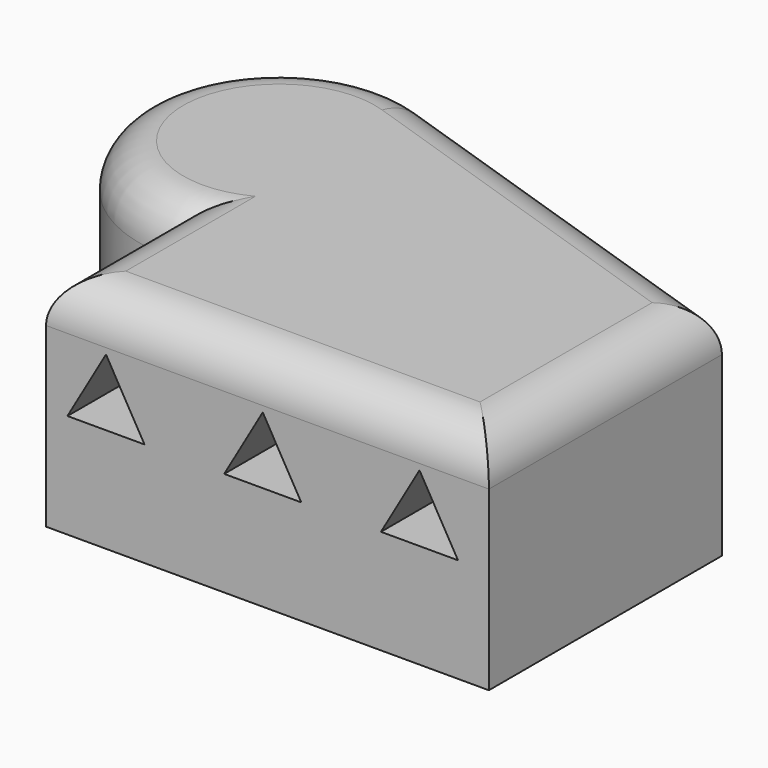
from build123d import *

# Parameters (mm, degrees)
F1_DEPTH = 25
F4_DEPTH = 25
F5_DEPTH = 23.7095438224
F6_R     = 5


# Not quite as in the source:
# - the program builds the solid bodies; features that only make, move or delete a surface that nothing else refers to are left out


with BuildPart() as f1:
    # F0 (on Top) → F1 (new body)
    with BuildSketch(Plane.XY):
        with BuildLine():
            ThreePointArc((-24.4463197887, 8.4633977604), (-29.1204506303, 19.7477478306), (-17.8361005601, 15.073616989))
            Line((-17.8361005601, 15.073616989), (-8.6304908186, 15.073616989))
            ThreePointArc((-8.6304908186, 15.073616989), (-11.6154192696, 24.3206942504), (-19.4435108685, 30.0773614855))
            ThreePointArc((-19.4435108685, 30.0773614855), (-40.0578075922, 17.607762717), (-24.4463197887, -0.7422119811))
            Line((-24.4463197887, -0.7422119811), (-24.4463197887, 8.4633977604))
        make_face()
        with BuildLine():
            Line((-17.8361005601, 15.073616989), (-24.4463197887, 15.073616989))
            Line((-24.4463197887, 15.073616989), (-24.4463197887, 8.4633977604))
            ThreePointArc((-24.4463197887, 8.4633977604), (-19.772188947, 10.3994861473), (-17.8361005601, 15.073616989))
        make_face()
        with BuildLine():
            Line((-24.4463197887, 8.4633977604), (-24.4463197887, 15.073616989))
            Line((-24.4463197887, 15.073616989), (-17.8361005601, 15.073616989))
            ThreePointArc((-17.8361005601, 15.073616989), (-29.1204506303, 19.7477478306), (-24.4463197887, 8.4633977604))
        make_face()
        with BuildLine():
            ThreePointArc((-19.4435108685, 30.0773614855), (-11.6154192696, 24.3206942504), (-8.6304908186, 15.073616989))
            Line((-8.6304908186, 15.073616989), (25.5536802113, 15.073616989))
            Line((25.5536802113, 15.073616989), (-19.4435108685, 30.0773614855))
        make_face()
        with BuildLine():
            Line((25.5536802113, 15.073616989), (-8.6304908186, 15.073616989))
            ThreePointArc((-8.6304908186, 15.073616989), (-13.2628398739, 3.8901370741), (-24.4463197887, -0.7422119811))
            Line((-24.4463197887, -0.7422119811), (-24.4463197887, -17.8190978634))
            Line((-24.4463197887, -17.8190978634), (25.5536802113, -17.8190978634))
            Line((25.5536802113, -17.8190978634), (25.5536802113, 15.073616989))
        make_face()
        with BuildLine():
            Line((-8.6304908186, 15.073616989), (-17.8361005601, 15.073616989))
            ThreePointArc((-17.8361005601, 15.073616989), (-19.772188947, 10.3994861473), (-24.4463197887, 8.4633977604))
            Line((-24.4463197887, 8.4633977604), (-24.4463197887, -0.7422119811))
            ThreePointArc((-24.4463197887, -0.7422119811), (-13.2628398739, 3.8901370741), (-8.6304908186, 15.073616989))
        make_face()
    extrude(amount=F1_DEPTH)

    # F3 (on face) → F4 (cut)
    with BuildSketch(Plane.XZ.offset(17.8190978634)):
        Polygon((-22.0338956294, 11.7883440107), (-13.3311382654, 11.7883440107), (-17.6825169474, 19.3251529709), align=None)
        Polygon((4.3688617346, 11.7883440107), (0.0174830526, 19.3251529709), (-4.3338956294, 11.7883440107), align=None)
        Polygon((22.0688617346, 11.7883440107), (17.7174830526, 19.3251529709), (13.3661043706, 11.7883440107), align=None)
    extrude(amount=-F4_DEPTH, mode=Mode.SUBTRACT)

    # F5 (cut, through all): faces of the model
    f5_faces = [f1.faces().sort_by_distance(p)[0] for p in [
        (-17.6825169474, 7.1809021366, 14.3006136641),
        (0.0174830526, 7.1809021366, 14.3006136641),
        (17.7174830526, 7.1809021366, 14.3006136641),
    ]]
    extrude(f5_faces, amount=-F5_DEPTH, mode=Mode.SUBTRACT)

    # F6
    f6_edges = [f1.edges().sort_by_distance(p)[0] for p in [
        (-40.057808, 17.607763, 25),
        (-24.44632, -9.280655, 25),
        (0.55368, -17.819098, 25),
        (25.55368, -1.37274, 25),
        (3.055085, 22.575489, 25),
    ]]
    fillet(f6_edges, radius=F6_R)


solid = f1.part
